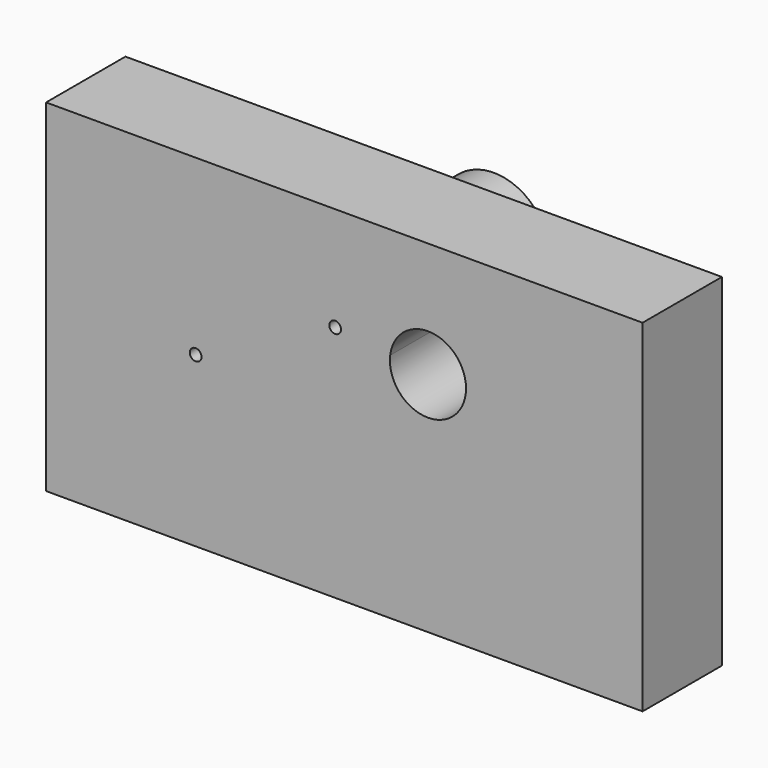
from build123d import *

# Parameters (mm, degrees)
F0_W     = 152.7194529772
F0_H     = 87.6065120101
F1_DEPTH = 25.4
F2_DEPTH = 25.4
F4_DEPTH = 25.4
F5_DEPTH = 25.4
F8_D     = 3
F9_D     = 3
F10_D    = 3
F11_D    = 3
F12_D    = 3


# Not quite as in the source:
# - a feature of the source that left no trace in its solid (it failed there, or was rolled back) is left out


with BuildPart() as f1:
    # F0 (on Front) → F1 (new body)
    with BuildSketch(Plane.XZ):
        with Locations((0.3946200013, -12.1346861124)):
            Rectangle(F0_W, F0_H)
        with BuildLine():
            ThreePointArc((-14.6484100073, -1.2818487871), (-12.6323252843, -6.8608521587), (-11.9481632112, -12.7533727135))
            ThreePointArc((-11.9481632112, -12.7533727135), (-62.6990011381, -18.6458932683), (-14.6484100073, -1.2818487871))
        make_face(mode=Mode.SUBTRACT)
        with BuildLine():
            ThreePointArc((12.1383150794, 3.3293733395), (0.4596359109, -8.9368839284), (-14.6484100073, -1.2818487871))
            ThreePointArc((-14.6484100073, -1.2818487871), (-5.1992136459, 18.8610416578), (12.2427693617, 5.0479834842))
            ThreePointArc((12.2427693617, 5.0479834842), (12.2166317196, 4.1870927352), (12.1383150794, 3.3293733395))
        make_face(mode=Mode.SUBTRACT)
        with BuildLine():
            ThreePointArc((31.5604166727, 2.1489301), (21.2221824249, -7.5800405103), (12.1383150794, 3.3293733395))
            ThreePointArc((12.1383150794, 3.3293733395), (22.4048039377, 11.8779007103), (31.5604166727, 2.1489301))
        make_face(mode=Mode.SUBTRACT)
        with BuildLine():
            ThreePointArc((-14.6484100073, -1.2818487871), (-62.6990011381, -18.6458932683), (-11.9481632112, -12.7533727135))
            ThreePointArc((-11.9481632112, -12.7533727135), (-12.6323252843, -6.8608521587), (-14.6484100073, -1.2818487871))
        make_face()
        with BuildLine():
            ThreePointArc((12.2427693617, 5.0479834842), (-5.1992136459, 18.8610416578), (-14.6484100073, -1.2818487871))
            ThreePointArc((-14.6484100073, -1.2818487871), (0.4596359109, -8.9368839284), (12.1383150794, 3.3293733395))
            ThreePointArc((12.1383150794, 3.3293733395), (12.2166317196, 4.1870927352), (12.2427693617, 5.0479834842))
        make_face()
    extrude(amount=F1_DEPTH)

    # F11 (through all)
    with Locations(Plane(origin=(0, 0, 0), x_dir=(1, 0, 0), z_dir=(0, 1, 0))):
        with Locations((-1.9478002292, -5.0479834842)):
            Hole(F11_D / 2)

    # F12 (through all)
    with Locations(Plane(origin=(0, 0, 0), x_dir=(1, 0, 0), z_dir=(0, 1, 0))):
        with Locations((-37.6656632112, 12.7533727135)):
            Hole(F12_D / 2)


with BuildPart() as f2:
    # F0 (on Front) → F2 (new body)
    with BuildSketch(Plane.XZ):
        with BuildLine():
            ThreePointArc((-14.6484100073, -1.2818487871), (-62.6990011381, -18.6458932683), (-11.9481632112, -12.7533727135))
            ThreePointArc((-11.9481632112, -12.7533727135), (-12.6323252843, -6.8608521587), (-14.6484100073, -1.2818487871))
        make_face()
    extrude(amount=-F2_DEPTH)

    # F10 (through all)
    with Locations(Plane.XZ):
        with Locations((-37.6656632112, -12.7533727135)):
            Hole(F10_D / 2)


with BuildPart() as f2b:
    # F0 (on Front) → F2, piece 2 (new body)
    with BuildSketch(Plane.XZ):
        with BuildLine():
            ThreePointArc((31.5604166727, 2.1489301), (22.4048039377, 11.8779007103), (12.1383150794, 3.3293733395))
            ThreePointArc((12.1383150794, 3.3293733395), (21.2221824249, -7.5800405103), (31.5604166727, 2.1489301))
        make_face()
    extrude(amount=-F2_DEPTH)

    # F8 (through all)
    with Locations(Plane.XZ):
        with Locations((21.8134931813, 2.1489301)):
            Hole(F8_D / 2)


with BuildPart() as f4:
    # F0 (on Front) → F4 (new body)
    with BuildSketch(Plane.XZ):
        with BuildLine():
            ThreePointArc((31.5604166727, 2.1489301), (22.4048039377, 11.8779007103), (12.1383150794, 3.3293733395))
            ThreePointArc((12.1383150794, 3.3293733395), (21.2221824249, -7.5800405103), (31.5604166727, 2.1489301))
        make_face()
    extrude(amount=F4_DEPTH)


with BuildPart() as f5:
    # F0 (on Front) → F5 (new body)
    with BuildSketch(Plane.XZ):
        with BuildLine():
            ThreePointArc((12.2427693617, 5.0479834842), (-5.1992136459, 18.8610416578), (-14.6484100073, -1.2818487871))
            ThreePointArc((-14.6484100073, -1.2818487871), (0.4596359109, -8.9368839284), (12.1383150794, 3.3293733395))
            ThreePointArc((12.1383150794, 3.3293733395), (12.2166317196, 4.1870927352), (12.2427693617, 5.0479834842))
        make_face()
    extrude(amount=-F5_DEPTH)

    # F9 (through all)
    with Locations(Plane.XZ):
        with Locations((-1.9478002292, 5.0479834842)):
            Hole(F9_D / 2)


solid = Compound([f1.part, f2.part, f2b.part, f5.part])
